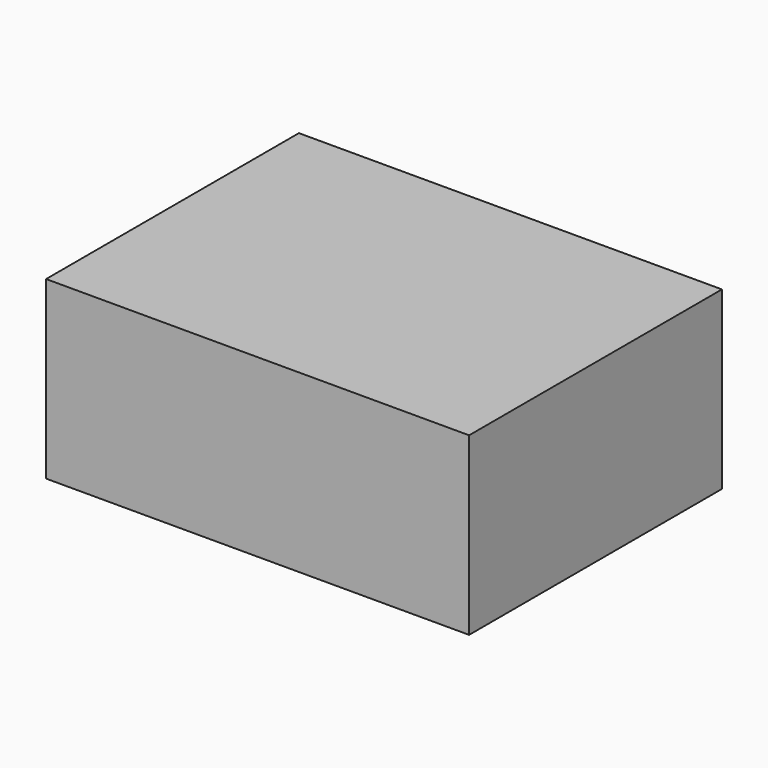
from build123d import *

# Parameters (mm, degrees)
F0_W     = 30.12
F0_H     = 22.5
F1_DEPTH = 11.01
F2_W     = 19.53
F2_H     = 11.91
F3_DEPTH = 6.01
F4_W     = 11
F4_H     = 6
F5_DEPTH = 1
F6_DEPTH = 1.5


with BuildPart() as f1:
    # F0 (on Top) → F1 (new body)
    with BuildSketch(Plane.XY):
        Rectangle(F0_W, F0_H)
    extrude(amount=-F1_DEPTH)

    # F2 (on face) → F3 (cut)
    with BuildSketch(Plane(origin=(0, 0, -11.01), x_dir=(1, 0, 0), z_dir=(0, 0, -1))):
        Rectangle(F2_W, F2_H)
    extrude(amount=-F3_DEPTH, mode=Mode.SUBTRACT)

    # F4 (on face) → F5 (cut)
    with BuildSketch(Plane(origin=(0, 0, -5), x_dir=(1, 0, 0), z_dir=(0, 0, -1))):
        Rectangle(F4_W, F4_H)
    extrude(amount=-F5_DEPTH, mode=Mode.SUBTRACT)

    # F6 (add): a face of the model
    f6_faces = [f1.faces().sort_by_distance(p)[0] for p in [
        (0, 0, 0),
    ]]
    extrude(f6_faces, amount=F6_DEPTH)


solid = f1.part
